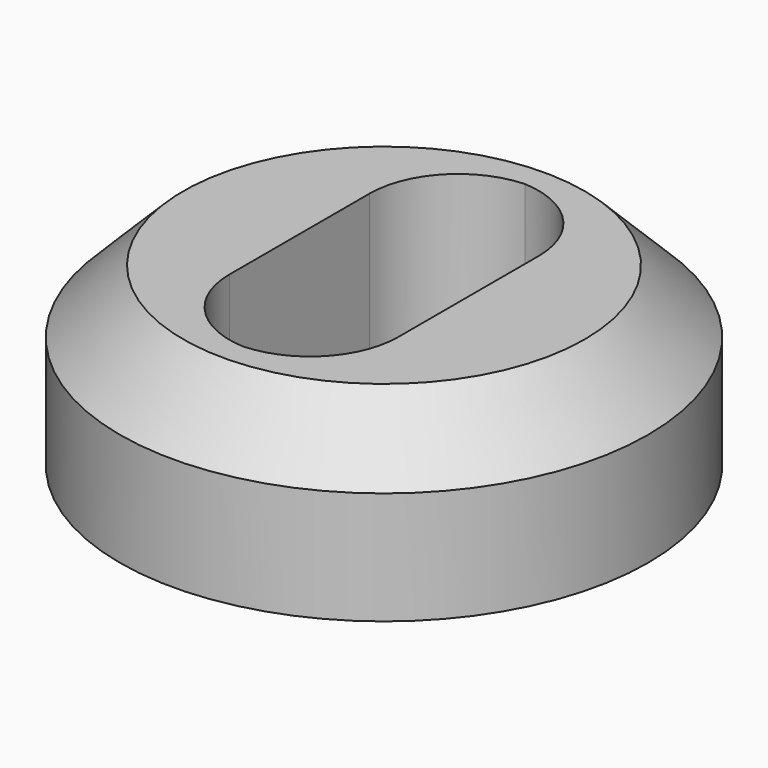
from build123d import *

# Parameters (mm, degrees)
F0_R        = 9.525
F0_W        = 6.096
F0_H        = 12.7
F1_DEPTH    = 6.35
F2_T1_DEPTH = 6.35
F3_SIZE     = 2.286


# Not quite as in the source:
# - a fillet or chamfer that OpenCascade refuses, or shapes differently, is made with other operations: its cross-section is extruded or revolved along the edge and cut away or added


with BuildPart() as f1:
    # F0 (on Top) → F1 (new body)
    with BuildSketch(Plane.XY):
        Circle(F0_R)
        Rectangle(F0_W, F0_H, mode=Mode.SUBTRACT)
    extrude(amount=F1_DEPTH)

    # F2: fillet of radius 3.1886932732 on 4 edges, made by hand

    # F2_s2 → F2_t1 (join)
    with BuildSketch(Plane.XY):
        with BuildLine():
            ThreePointArc((0.1406932732, 6.35), (-2.1140533634, 5.4160533634), (-3.048, 3.1613067268))
            Line((-3.048, 3.1613067268), (-3.048, 6.35))
            Line((-3.048, 6.35), (0.1406932732, 6.35))
        make_face()
        with BuildLine():
            ThreePointArc((-0.1406932732, 6.35), (2.1140533634, 5.4160533634), (3.048, 3.1613067268))
            Line((3.048, 3.1613067268), (3.048, 6.35))
            Line((3.048, 6.35), (-0.1406932732, 6.35))
        make_face()
        with BuildLine():
            ThreePointArc((0.1406932732, -6.35), (-2.1140533634, -5.4160533634), (-3.048, -3.1613067268))
            Line((-3.048, -3.1613067268), (-3.048, -6.35))
            Line((-3.048, -6.35), (0.1406932732, -6.35))
        make_face()
        with BuildLine():
            ThreePointArc((3.048, -3.1613067268), (2.1140533634, -5.4160533634), (-0.1406932732, -6.35))
            Line((-0.1406932732, -6.35), (3.048, -6.35))
            Line((3.048, -6.35), (3.048, -3.1613067268))
        make_face()
    extrude(amount=F2_T1_DEPTH)

    # F3
    f3_edges = [f1.edges().sort_by_distance(p)[0] for p in [
        (-9.525, 0, 6.35),
    ]]
    chamfer(f3_edges, length=F3_SIZE)


solid = f1.part
